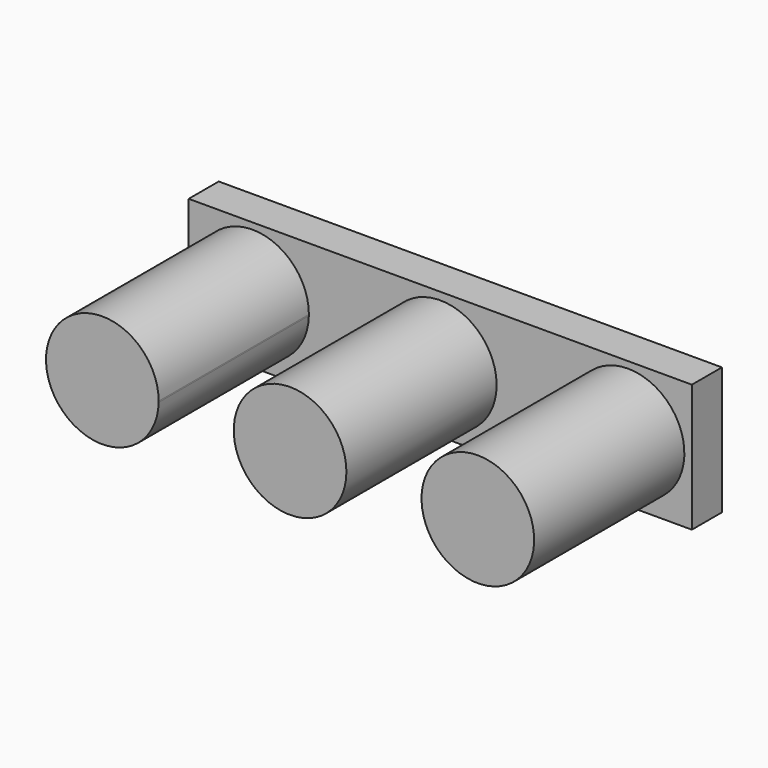
from build123d import *

# Parameters (mm, degrees)
F0_W     = 67
F0_H     = 17
F1_DEPTH = 5
F2_DEPTH = 30
F3_DEPTH = 30


with BuildPart() as f1:
    # F0 (on Front) → F1 (new body)
    with BuildSketch(Plane.XZ):
        Rectangle(F0_W, F0_H)
        with BuildLine():
            ThreePointArc((-17.498445447, 0.1526953798), (-17.4988340953, 0.0763437334), (-17.5, 0))
            ThreePointArc((-17.5, 0), (-32.4980567986, 0.2290470263), (-17.498445447, 0.1526953798))
        make_face(mode=Mode.SUBTRACT)
        with BuildLine():
            ThreePointArc((-7.5, 0), (0, 7.5), (7.5, 0))
            ThreePointArc((7.5, 0), (0, -7.5), (-7.5, 0))
        make_face(mode=Mode.SUBTRACT)
        with BuildLine():
            ThreePointArc((32.4989989183, 0.1225366207), (25.0602692732, -7.3772131047), (17.5, 0))
            ThreePointArc((17.5, 0), (24.9377285633, 7.6222863461), (32.4989989183, 0.1225366207))
        make_face(mode=Mode.SUBTRACT)
    extrude(amount=F1_DEPTH)

    # F0 (on Front) → F2 (join)
    with BuildSketch(Plane.XZ):
        with BuildLine():
            ThreePointArc((-17.498445447, 0.1526953798), (-32.4980567986, 0.2290470263), (-17.5, 0))
            ThreePointArc((-17.5, 0), (-17.4988340953, 0.0763437334), (-17.498445447, 0.1526953798))
        make_face()
    extrude(amount=F2_DEPTH)

    # F0 (on Front) → F3 (join)
    with BuildSketch(Plane.XZ):
        with BuildLine():
            ThreePointArc((-7.5, 0), (0, -7.5), (7.5, 0))
            ThreePointArc((7.5, 0), (0, 7.5), (-7.5, 0))
        make_face()
        with BuildLine():
            ThreePointArc((32.4989989183, 0.1225366207), (24.9377285633, 7.6222863461), (17.5, 0))
            ThreePointArc((17.5, 0), (25.0602692732, -7.3772131047), (32.4989989183, 0.1225366207))
        make_face()
    extrude(amount=F3_DEPTH)


solid = f1.part
